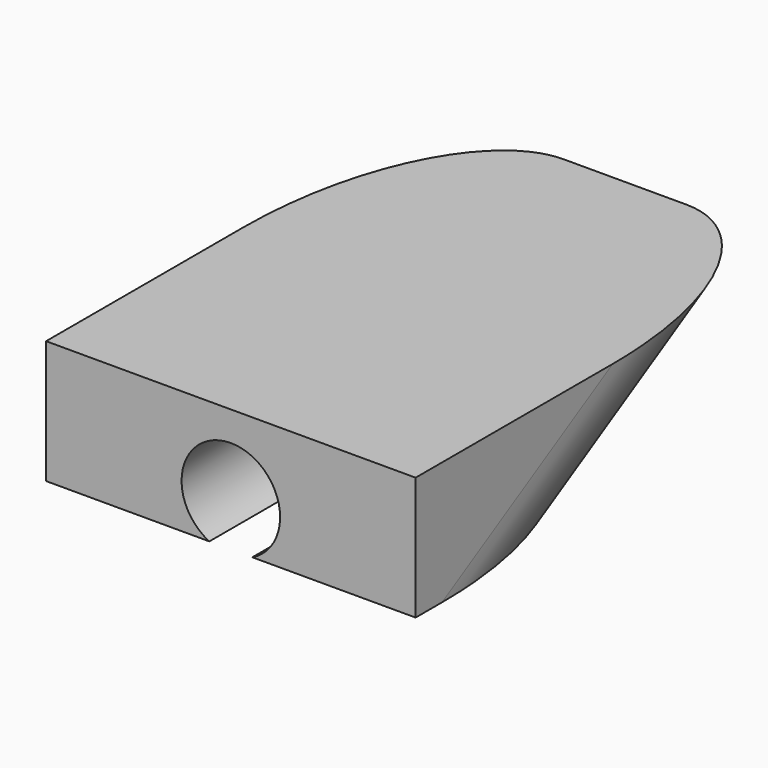
from build123d import *

# Parameters (mm, degrees)
F1_DEPTH = 10
F3_DEPTH = 10
F4_SIZE2 = 8.660244
F4_SIZE  = 4.99999
F5_R     = 5


# Not quite as in the source:
# - a fillet or chamfer is up to 0.001 mm smaller than in the source, because OpenCascade refuses the exact size


with BuildPart() as f1:
    # F0 (on Front) → F1 (new body)
    with BuildSketch(Plane.XZ):
        with BuildLine():
            Line((0.8717797887, -2.5), (7.5, -2.5))
            Line((7.5, -2.5), (7.5, 2.5))
            Line((7.5, 2.5), (-7.5, 2.5))
            Line((-7.5, 2.5), (-7.5, -2.5))
            Line((-7.5, -2.5), (-0.8717797887, -2.5))
            ThreePointArc((-0.8717797887, -2.5), (0, 1.3), (0.8717797887, -2.5))
        make_face()
    extrude(amount=F1_DEPTH)

    # F2 (on face) → F3 (join)
    with BuildSketch(Plane(origin=(0, 0, 0), x_dir=(-1, 0, 0), z_dir=(0, 1, 0))):
        with BuildLine():
            ThreePointArc((0.8717797887, -2.5), (0, 1.3), (-0.8717797887, -2.5))
            Line((-0.8717797887, -2.5), (0.8717797887, -2.5))
        make_face()
        with BuildLine():
            Line((7.5, 2.5), (-7.5, 2.5))
            Line((-7.5, 2.5), (-7.5, -2.5))
            Line((-7.5, -2.5), (-0.8717797887, -2.5))
            ThreePointArc((-0.8717797887, -2.5), (0, 1.3), (0.8717797887, -2.5))
            Line((0.8717797887, -2.5), (7.5, -2.5))
            Line((7.5, -2.5), (7.5, 2.5))
        make_face()
    extrude(amount=F3_DEPTH)

    # F4 (size 5 and 8.6602540378 in the source; OpenCascade refuses exactly that, so slightly less here)
    f4_edges = [f1.edges().sort_by_distance(p)[0] for p in [
        (0, 10, -2.5),
    ]]
    f4_side = f1.faces().sort_by_distance((0, 10, 0))[0]
    chamfer(f4_edges, length=F4_SIZE, length2=F4_SIZE2, reference=f4_side)

    # F5
    f5_edges = [f1.edges().sort_by_distance(p)[0] for p in [
        (0, 1.339756, -2.5),
        (7.5, 5.669878, -5e-06),
        (-7.5, 5.669878, -5e-06),
    ]]
    fillet(f5_edges, radius=F5_R)


solid = f1.part
